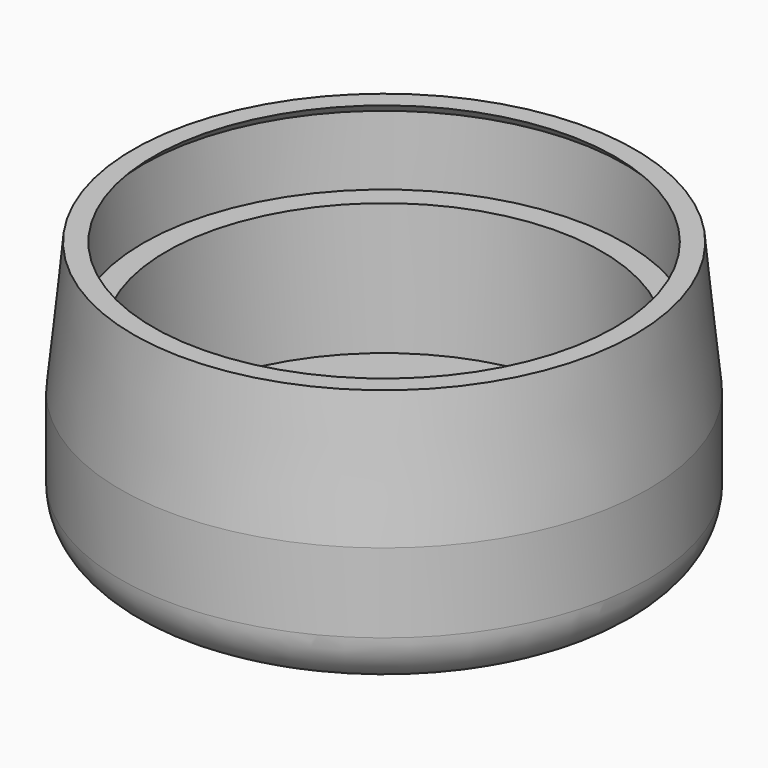
from build123d import *

# Parameters (mm, degrees)
F0_R        = 10
F1_DEPTH    = 10
F2_R        = 8.25
F3_DEPTH    = 8
F4_R        = 9.125
F4_R_2      = 8.25
F5_DEPTH    = 3
F6_R        = 9.125
F6_R_2      = 8.75
F7_DEPTH    = 1
F8_R        = 2
F9_S5_R     = 9.125
F9_T6_DEPTH = 15
F10_SIZE2   = 5
F10_SIZE    = 0.5


# Not quite as in the source:
# - a fillet or chamfer that OpenCascade refuses, or shapes differently, is made with other operations: its cross-section is extruded or revolved along the edge and cut away or added


with BuildPart() as f1:
    # F0 (on Top) → F1 (new body)
    with BuildSketch(Plane.XY):
        Circle(F0_R)
    extrude(amount=F1_DEPTH)

    # F2 (on face) → F3 (cut)
    with BuildSketch(Plane.XY.offset(10)):
        Circle(F2_R)
    extrude(amount=-F3_DEPTH, mode=Mode.SUBTRACT)

    # F4 (on face) → F5 (cut)
    with BuildSketch(Plane.XY.offset(10)):
        Circle(F4_R)
        Circle(F4_R_2, mode=Mode.SUBTRACT)
    extrude(amount=-F5_DEPTH, mode=Mode.SUBTRACT)

    # F6 (on face) → F7 (join)
    with BuildSketch(Plane.XY.offset(10)):
        Circle(F6_R)
        Circle(F6_R_2, mode=Mode.SUBTRACT)
    extrude(amount=-F7_DEPTH)

    # F8
    f8_edges = [f1.edges().sort_by_distance(p)[0] for p in [
        (-10, 0, 0),
    ]]
    fillet(f8_edges, radius=F8_R)

    # F9: chamfer of 1 on 1 edges, made by hand


with BuildPart() as f9_tool2:
    # F9_s3 → F9_t4 (revolve)
    with BuildSketch(Plane.XZ):
        Polygon((8.75, 10), (9.75, 9), (8.75, 9), align=None)
    revolve(axis=Axis((0, 0, 9), (0, 0, 1)))

    # F9_s5 → F9_t6 (intersect, symmetric)
    with BuildSketch(Plane.XY.offset(9.5)):
        Circle(F9_S5_R)
    extrude(amount=F9_T6_DEPTH, both=True, mode=Mode.INTERSECT)


with BuildPart() as f1_1:
    add(f1.part)

    # F9_t1: cut F9_tool2
    add(f9_tool2.part, mode=Mode.SUBTRACT)

    # F10
    f10_edges = [f1_1.edges().sort_by_distance(p)[0] for p in [
        (-10, 0, 10),
    ]]
    f10_side = f1_1.faces().sort_by_distance((-9.717157, 0, 10))[0]
    chamfer(f10_edges, length=F10_SIZE, length2=F10_SIZE2, reference=f10_side)


solid = f1_1.part
